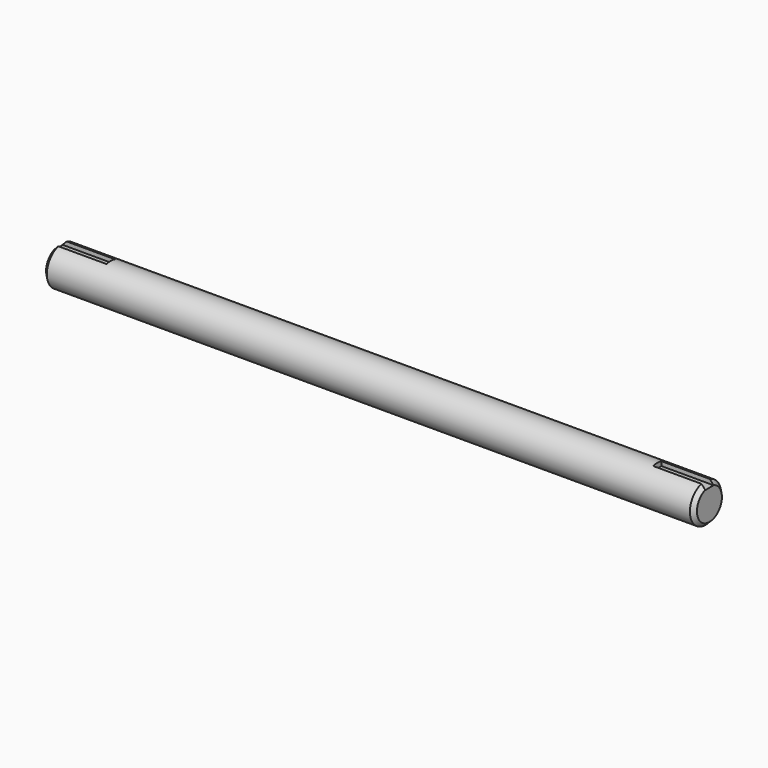
from build123d import *

# Parameters (mm, degrees)
F0_W     = 500
F0_H     = 15
F3_DEPTH = 40
F4_SIZE2 = 3
F4_SIZE  = 3


# Not quite as in the source:
# - a pattern or mirror of a feature is missing from the dataset's text; its kind, count and spacing are read off the source's solid


with BuildPart() as f1:
    # F0 (on Top) → F1 (revolve)
    with BuildSketch(Plane.XY):
        with Locations((0, 7.5)):
            Rectangle(F0_W, F0_H)
    revolve(axis=Axis((0, 0, 0), (1, 0, 0)))

    # F2 (on face) → F3 (cut)
    with BuildSketch(Plane.YZ.offset(250)):
        with BuildLine():
            ThreePointArc((4, 14.4568322948), (0, 15), (-4, 14.4568322948))
            Line((-4, 14.4568322948), (-4, 11.1568322948))
            Line((-4, 11.1568322948), (4, 11.1568322948))
            Line((4, 11.1568322948), (4, 14.4568322948))
        make_face()
    f3 = extrude(amount=-F3_DEPTH, mode=Mode.SUBTRACT)

    # F3_copies: F3 across plane
    add(f3.mirror(Plane(origin=(0, 0, 0), x_dir=(0, 0, -1), z_dir=(-1, 0, 0))), mode=Mode.SUBTRACT)

    # F4
    f4_edges = [f1.edges().sort_by_distance(p)[0] for p in [
        (250, -9.082951, -11.937336),
        (250, 11.937336, 9.082951),
        (-250, 11.937336, 9.082951),
        (-250, -9.082951, -11.937336),
    ]]
    chamfer(f4_edges, length=F4_SIZE, length2=F4_SIZE2)


solid = f1.part
